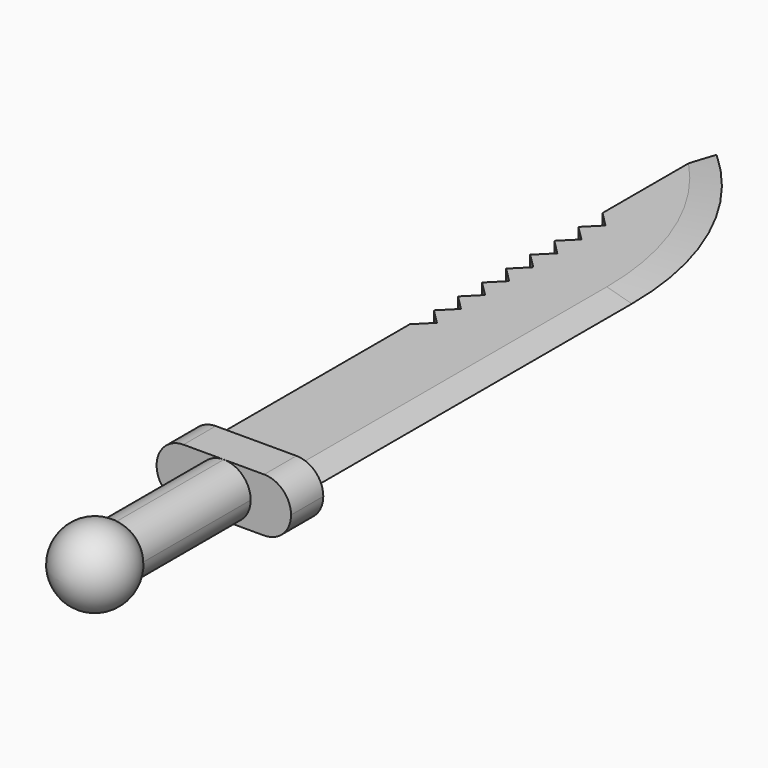
from build123d import *

# Parameters (mm, degrees)
F1_DEPTH    = 304.8
F2_T1_DEPTH = 574.3112662849
F3_T1_DEPTH = 224.1861106845
F3_T4_ANGLE = 60.5895449389
F3_T6_ANGLE = 60.5895449389
F5_DEPTH    = 19.05
F7_DEPTH    = 63.5
F8_R        = 12.69999
F12_DEPTH   = 25.4


# Not quite as in the source:
# - a fillet or chamfer that OpenCascade refuses, or shapes differently, is made with other operations: its cross-section is extruded or revolved along the edge and cut away or added
# - a fillet or chamfer is up to 0.001 mm smaller than in the source, because OpenCascade refuses the exact size


with BuildPart() as f1:
    # F0 (on Front) → F1 (new body)
    with BuildSketch(Plane.XZ):
        Polygon((-25.4, 0), (0, 0), (25.4, 0), (25.4, 3.175), (-25.4, 3.175), align=None)
        Polygon((25.4, 0), (0, 0), (-25.4, 0), (-25.4, -3.175), (25.4, -3.175), align=None)
    extrude(amount=-F1_DEPTH)

    # F2: fillet of radius 152.4 on 1 edges, made by hand

    # F2_s2 → F2_t1 (cut)
    with BuildSketch(Plane.XY.offset(-287.1556331425)):
        with BuildLine():
            ThreePointArc((25.4, 191.207746743), (12.1215296063, 253.4247862097), (-25.4, 304.8))
            Line((-25.4, 304.8), (25.4, 304.8))
            Line((25.4, 304.8), (25.4, 191.207746743))
        make_face()
    extrude(amount=F2_T1_DEPTH, mode=Mode.SUBTRACT)

    # F3: chamfer of 12.7 x 3.4029547439 on 4 edges, made by hand

    # F3_s2 → F3_t1 (cut)
    with BuildSketch(Plane.XZ.offset(-191.207746743)):
        Polygon((12.7, 3.175), (25.4, -0.2279547439), (25.4, 3.175), align=None)
        Polygon((25.4, 0.2279547439), (12.7, -3.175), (25.4, -3.175), align=None)
    extrude(amount=F3_T1_DEPTH, mode=Mode.SUBTRACT)

    # F3_s3 → F3_t4 (revolve, cut)
    with BuildSketch(Plane(origin=(-178.1690956727, 100.4359641468, 0), x_dir=(0, 0, 1), z_dir=(-0.8711242188, 0.4910627204, 0))):
        Polygon((3.175, 243.9007335274), (-0.2279547439, 256.6007335274), (3.175, 256.6007335274), align=None)
    revolve(axis=Axis((-127.0000000001, 191.207746743, 3.175), (0, 0, -1)), revolution_arc=F3_T4_ANGLE, mode=Mode.SUBTRACT)

    # F3_s5 → F3_t6 (revolve, cut)
    with BuildSketch(Plane(origin=(-178.1690956727, 100.4359641468, 0), x_dir=(0, 0, 1), z_dir=(-0.8711242188, 0.4910627204, 0))):
        Polygon((0.2279547439, 256.6007335274), (-3.175, 243.9007335274), (-3.175, 256.6007335274), align=None)
    revolve(axis=Axis((-127.0000000001, 191.207746743, -3.175), (0, 0, -1)), revolution_arc=F3_T6_ANGLE, mode=Mode.SUBTRACT)

    # F4 (on face) → F5 (join)
    with BuildSketch(Plane.XZ):
        Polygon((31.75, 12.7), (0, 12.7), (-31.75, 12.7), (-31.75, -12.7), (0, -12.7), (31.75, -12.7), align=None)
        Polygon((-25.4, 3.175), (0, 3.175), (12.7, 3.175), (24.5492613139, 0), (12.7, -3.175), (-25.4, -3.175), align=None, mode=Mode.SUBTRACT)
        Polygon((12.7, 3.175), (0, 3.175), (-25.4, 3.175), (-25.4, -3.175), (12.7, -3.175), (24.5492613139, 0), align=None)
    extrude(amount=F5_DEPTH)

    # F6 (on face) → F7 (join)
    with BuildSketch(Plane.XZ.offset(19.05)):
        with BuildLine():
            ThreePointArc((0, -12.7), (8.9802561211, -8.9802561211), (12.7, 0))
            ThreePointArc((12.7, 0), (8.980256117, 8.9802561251), (-1.15e-08, 12.7))
            ThreePointArc((-1.15e-08, 12.7), (-12.7, -5.7e-09), (0, -12.7))
        make_face()
    extrude(amount=F7_DEPTH)

    # F8 (radius 12.7 in the source; OpenCascade refuses exactly that, so slightly less here)
    f8_edges = [f1.edges().sort_by_distance(p)[0] for p in [
        (-31.75, -9.525, 12.7),
        (31.75, -9.525, 12.7),
        (31.75, -9.525, -12.7),
        (-31.75, -9.525, -12.7),
    ]]
    fillet(f8_edges, radius=F8_R)

    # F11 (on face) → F12 (cut)
    with BuildSketch(Plane.XY.offset(3.175)):
        Polygon((-18.2896524204, 229.1802964913), (-25.4, 236.2906440709), (-25.4, 222.0699489117), align=None)
        Polygon((-18.2896524204, 214.959601332), (-25.4, 222.0699489117), (-25.4, 207.8492537524), align=None)
        Polygon((-18.2896524204, 200.7389061727), (-25.4, 207.8492537524), (-25.4, 193.6285585931), align=None)
        Polygon((-18.2896524204, 186.5182110135), (-25.4, 193.6285585931), (-25.4, 179.4078634338), align=None)
        Polygon((-18.2896524204, 172.2975158542), (-25.4, 179.4078634338), (-25.4, 165.1871682745), align=None)
        Polygon((-18.2896524204, 158.0768206949), (-25.4, 165.1871682745), (-25.4, 150.9664731153), align=None)
        Polygon((-25.4, 150.9664731153), (-25.4, 136.745777956), (-18.2896524204, 143.8561255356), align=None)
        Polygon((-25.4, 136.745777956), (-25.4, 122.5250827967), (-18.2896524204, 129.6354303763), align=None)
    extrude(amount=-F12_DEPTH, mode=Mode.SUBTRACT)


with BuildPart() as f10:
    # F9 (on Top) → F10 (revolve)
    with BuildSketch(Plane.XY):
        with BuildLine():
            Line((0, -113.2105122421), (0, -82.55))
            Line((0, -82.55), (-12.7, -82.55))
            ThreePointArc((-12.7, -82.55), (-16.5933496539, -102.1231904719), (0, -113.2105122421))
        make_face()
    revolve(axis=Axis((0, -97.8802561211, 0), (0, -1, 0)))


solid = Compound([f1.part, f10.part])
